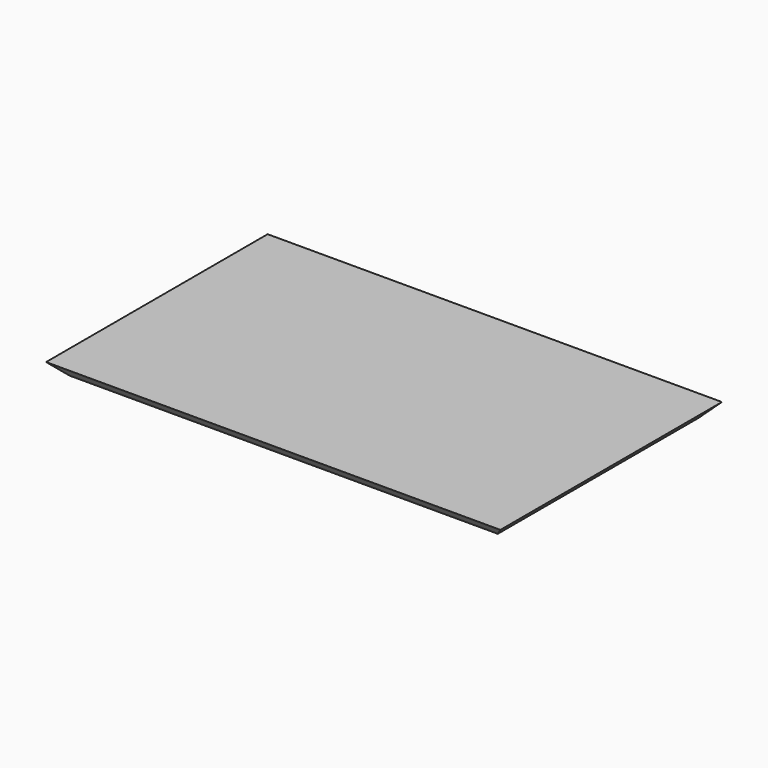
from build123d import *

# Parameters (mm, degrees)
F1_DEPTH = 406.4
F2_SIZE  = 19.04999
F3_SIZE  = 19.04999


# Not quite as in the source:
# - a fillet or chamfer is up to 0.001 mm smaller than in the source, because OpenCascade refuses the exact size


with BuildPart() as f1:
    # F0 (on Front) → F1 (new body)
    with BuildSketch(Plane.XZ):
        Polygon((333.375, 9.525), (-333.375, 9.525), (-314.325, -9.525), (314.325, -9.525), align=None)
    extrude(amount=-F1_DEPTH)

    # F2 (size 19.05 in the source; OpenCascade refuses exactly that, so slightly less here)
    f2_edges = [f1.edges().sort_by_distance(p)[0] for p in [
        (0, 406.4, -9.525),
    ]]
    chamfer(f2_edges, length=F2_SIZE)

    # F3 (size 19.05 in the source; OpenCascade refuses exactly that, so slightly less here)
    f3_edges = [f1.edges().sort_by_distance(p)[0] for p in [
        (0, 0, -9.525),
    ]]
    chamfer(f3_edges, length=F3_SIZE)


solid = f1.part
